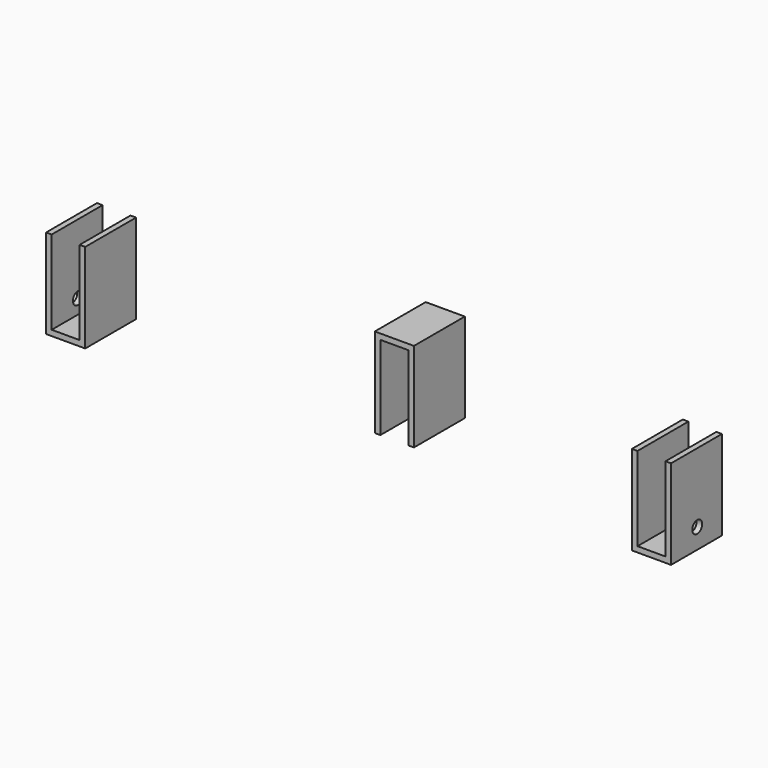
from build123d import *

# Parameters (mm, degrees)
F1_W      = 14
F1_H      = 22.75
F2_DEPTH  = 2
F3_W      = 2
F3_H      = 22.75
F4_DEPTH  = 30
F5_R      = 2.2
F6_DEPTH  = 2
F7_R      = 2.2
F8_DEPTH  = 2
F10_ANGLE = 180
F13_W     = 7.1573019959
F13_H     = 10.3748198599
F14_DEPTH = 2
F16_W     = 18.6804127879
F16_H     = 9.1584324837
F17_DEPTH = 2


with BuildPart() as f2:
    # F1 (on Top) → F2 (new body)
    with BuildSketch(Plane.XY):
        with Locations((104.7940782905, -32.9721670151)):
            Rectangle(F1_W, F1_H)
    extrude(amount=F2_DEPTH)

    # F3 (on face) → F4 (join)
    with BuildSketch(Plane.XY.offset(2)):
        with Locations((98.7940782905, -32.9721670151)):
            Rectangle(F3_W, F3_H)
        with Locations((110.7940782905, -32.9721670151)):
            Rectangle(F3_W, F3_H)
    extrude(amount=F4_DEPTH)

    # F5 (on face) → F6 (cut, through all)
    with BuildSketch(Plane.YZ.offset(111.7940782905)):
        with Locations((-32.6319672167, 7.209660951)):
            Circle(F5_R)
    extrude(amount=-F6_DEPTH, mode=Mode.SUBTRACT)

    # F7 (on face) → F8 (cut, through all)
    with BuildSketch(Plane.XY.offset(2)):
        with Locations((104.3131947517, -33.9013487101)):
            Circle(F7_R)
    extrude(amount=-F8_DEPTH, mode=Mode.SUBTRACT)


with BuildPart() as f9_1:
    # F9: instance of F2
    add(f2.part.mirror(Plane.YZ))


with BuildPart() as f10_1:
    # F10: copy of F9_1
    add(f9_1.part.rotate(Axis((-97.7940782905, -32.9721670151, 0), (0, 1, 0)), F10_ANGLE))


with BuildPart() as f10_1_1:
    # F11: moved
    add(f10_1.part.moved(Location((90.8, 16, 28.4))))

    # F13 (on offset) → F14 (join, through all)
    with BuildSketch(Plane.XY.offset(28.4)):
        with Locations((-0.1049609855, -17.7491279319)):
            Rectangle(F13_W, F13_H)
    extrude(amount=-F14_DEPTH)

    # F16 (on offset) → F17 (join, through all)
    with BuildSketch(Plane.YZ.offset(7.0059217095)):
        with Locations((-16.3181161042, 20.9184978157)):
            Rectangle(F16_W, F16_H)
    extrude(amount=-F17_DEPTH)


solid = Compound([f2.part, f9_1.part, f10_1_1.part])
